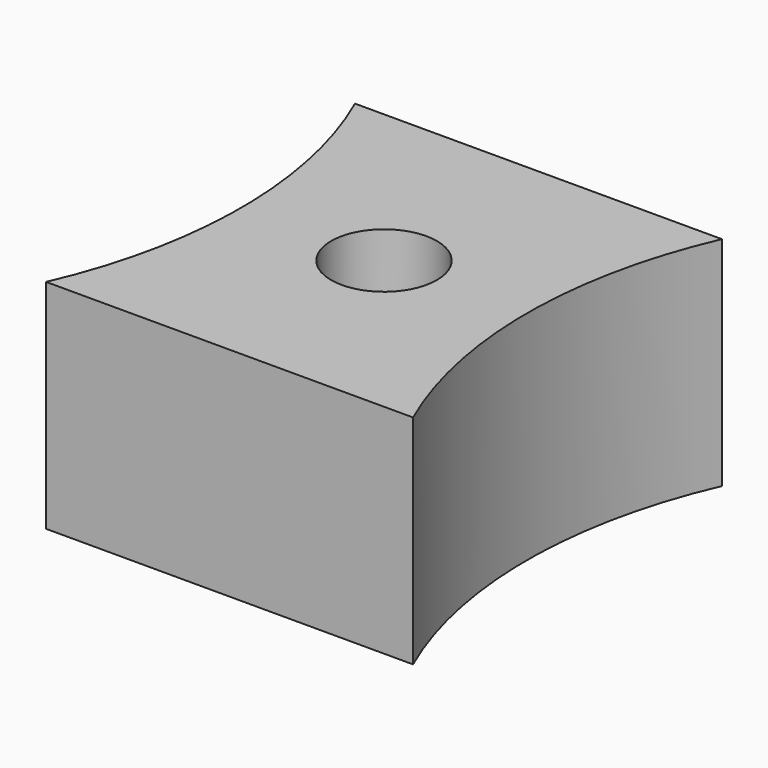
from build123d import *

# Parameters (mm, degrees)
F0_R     = 10
F1_DEPTH = 41.1


# Not quite as in the source:
# - a feature names something its author has since deleted; it is built from what else it names


with BuildPart() as f1:
    # F0 (on Top) → F1 (new body)
    with BuildSketch(Plane.XY):
        with BuildLine():
            ThreePointArc((-34.6869575489, 36.5), (-27, 0), (-34.6869575489, -36.5))
            Line((-34.6869575489, -36.5), (34.6869575489, -36.5))
            ThreePointArc((34.6869575489, -36.5), (27, 0), (34.6869575489, 36.5))
            Line((34.6869575489, 36.5), (-34.6869575489, 36.5))
        make_face()
        Circle(F0_R, mode=Mode.SUBTRACT)
    extrude(amount=F1_DEPTH)


solid = f1.part
